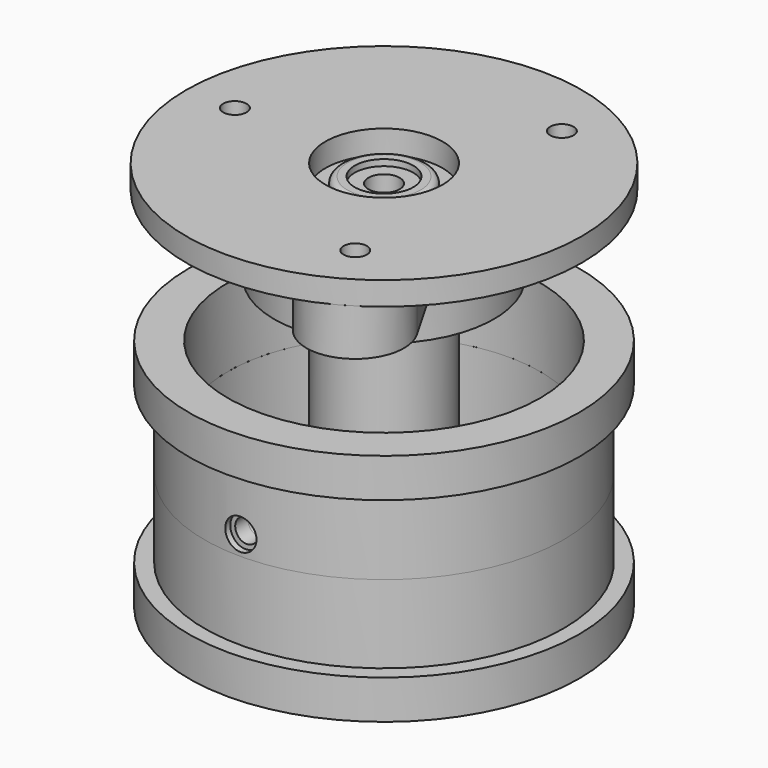
from build123d import *

# Parameters (mm, degrees)
F4_R           = 7.5
F4_R_2         = 3.75
F4_R_3         = 2.25
F5_DEPTH       = 10
F6_DEPTH       = 7.5
F9_W           = 2.45
F9_H           = 5
F11_R          = 0.2
F11_2_R        = 0.2
F12_R          = 0.6
F12_2_R        = 0.6
F13_R          = 0.8
F18_R          = 3.75
F18_R_2        = 2
F19_DEPTH      = 2
F20_DEPTH      = 6
F22_COUNT      = 3
F2_W           = 2
F2_H           = 5
F27_R          = 1.5
F28_REACH      = 54.2436406871
F31_END_RADIUS = 20
F30_R          = 3.5
F30_R_2        = 1.5
F31_REACH      = 16.9004949366
F27_R_2        = 2
F35_R          = 2
F36_DEPTH      = 47.1000001314
F38_DEPTH      = 4
F41_DEPTH      = 1
F43_R          = 25.35
F43_R_2        = 2
F43_R_3        = 7.5
F43_R_4        = 1.5
F44_DEPTH      = 3


with BuildPart() as f5:
    # F4 (on Top) → F5 (new body)
    with BuildSketch(Plane.XY):
        Circle(F4_R)
        Circle(F4_R_2, mode=Mode.SUBTRACT)
        Circle(F4_R_2)
        Circle(F4_R_3, mode=Mode.SUBTRACT)
    extrude(amount=F5_DEPTH)

    # F4 (on Top) → F6 (cut)
    with BuildSketch(Plane.XY):
        Circle(F4_R_2)
        Circle(F4_R_3, mode=Mode.SUBTRACT)
    extrude(amount=F6_DEPTH, mode=Mode.SUBTRACT)

    # F7 (on Front) → F8 (revolve)
    with BuildSketch(Plane.XZ):
        Polygon((-4.875, 12), (-6.0297005384, 10), (-3.7202994616, 10), align=None)
    revolve(axis=Axis((0, 0, 0), (0, 0, -1)))

    # F11
    f11_edges = [f5.edges().sort_by_distance(p)[0] for p in [
        (4.875, 0, 12),
    ]]
    fillet(f11_edges, radius=F11_R)

    # F12
    f12_edges = [f5.edges().sort_by_distance(p)[0] for p in [
        (-2.25, 0, 7.5),
        (-3.75, 0, 7.5),
    ]]
    fillet(f12_edges, radius=F12_R)



with BuildPart() as f10:
    # F9 (on Front) → F10 (revolve)
    with BuildSketch(Plane.XZ):
        Polygon((1.5, 20), (1.5, 10), (3.6048294078, 10), (4.875, 12.2), (6.1451705922, 10), (7.5, 10), (7.5, 35.7358983849), (5.5, 39.2), (5.5, 40), (3.95, 40), (1.5, 40), (1.5, 37), (0, 37), (0, 20), align=None)
        with Locations((2.725, 42.5)):
            Rectangle(F9_W, F9_H)
    revolve(axis=Axis((0, 0, 27.5), (0, 0, 1)))

    # F11#2
    f11_2_edges = [f10.edges().sort_by_distance(p)[0] for p in [
        (-4.875, 0, 12.2),
    ]]
    fillet(f11_2_edges, radius=F11_2_R)

    # F12#2
    f12_2_edges = [f10.edges().sort_by_distance(p)[0] for p in [
        (-1.5, 0, 20),
    ]]
    fillet(f12_2_edges, radius=F12_2_R)


with BuildPart() as f10b:
    # F9 (on Front) → F10, piece 2 (revolve)
    with BuildSketch(Plane.XZ):
        Polygon((2, 45.2), (3.95, 45.2), (3.95, 47), (5.5, 47), (5.5, 48.5), (3.75, 48.5), (3.75, 47.7), (2, 47.7), align=None)
    revolve(axis=Axis((0, 0, 27.5), (0, 0, 1)))

    # F13
    f13_edges = [f10b.edges().sort_by_distance(p)[0] for p in [
        (-5.5, 0, 48.5),
    ]]
    fillet(f13_edges, radius=F13_R)


with BuildPart() as f15:
    # F14 (on Front) → F15 (revolve)
    with BuildSketch(Plane.XZ):
        Polygon((-5.5, 40), (-5.5, 47), (-11, 47), (-11, 43.5), (-11, 40), align=None)
        Polygon((-4, 47), (-5.5, 47), (-5.5, 40), (-4, 40), (-4, 43.5), align=None)
    revolve(axis=Axis((0, 0, 43.5), (0, 0, 1)))


with BuildPart() as f17:
    # F16 (on Front) → F17 (revolve)
    with BuildSketch(Plane.XZ):
        Polygon((-7, 38.5), (-7, 40), (-11.1, 40), (-11.1, 47), (-14.1, 47), (-14.1, 44), (-14.1, 37), (-7.8660254038, 37), align=None)
    revolve(axis=Axis((0, 0, 42.5), (0, 0, -1)))

    # F18 (on face) → F19 (join)
    with BuildSketch(Plane.XY.offset(47)):
        with BuildLine():
            ThreePointArc((-13.7318717277, 3.2008903219), (-16.0131783751, 5.4345222657), (-19.1, 6.25))
            ThreePointArc((-19.1, 6.25), (-25.35, 0), (-19.1, -6.25))
            ThreePointArc((-19.1, -6.25), (-16.0131783751, -5.4345222657), (-13.7318717277, -3.2008903219))
            ThreePointArc((-13.7318717277, -3.2008903219), (-14.1, 0), (-13.7318717277, 3.2008903219))
        make_face()
        with Locations((-19.1, 0)):
            Circle(F18_R, mode=Mode.SUBTRACT)
        with Locations((-19.1, 0)):
            Circle(F18_R)
        with Locations((-19.1, 0)):
            Circle(F18_R_2, mode=Mode.SUBTRACT)
        with BuildLine():
            ThreePointArc((-13.7318717277, -3.2008903219), (-16.0131783751, -5.4345222657), (-19.1, -6.25))
            Line((-19.1, -6.25), (-12.6391257609, -6.25))
            ThreePointArc((-12.6391257609, -6.25), (-13.2733433842, -4.756927097), (-13.7318717277, -3.2008903219))
        make_face()
        with BuildLine():
            Line((-12.6391257609, 6.25), (-19.1, 6.25))
            ThreePointArc((-19.1, 6.25), (-16.0131783751, 5.4345222657), (-13.7318717277, 3.2008903219))
            ThreePointArc((-13.7318717277, 3.2008903219), (-13.2733433842, 4.756927097), (-12.6391257609, 6.25))
        make_face()
    extrude(amount=-F19_DEPTH)

    # F18 (on face) → F20 (join)
    with BuildSketch(Plane.XY.offset(47)):
        with BuildLine():
            ThreePointArc((-13.7318717277, 3.2008903219), (-16.0131783751, 5.4345222657), (-19.1, 6.25))
            ThreePointArc((-19.1, 6.25), (-25.35, 0), (-19.1, -6.25))
            ThreePointArc((-19.1, -6.25), (-16.0131783751, -5.4345222657), (-13.7318717277, -3.2008903219))
            ThreePointArc((-13.7318717277, -3.2008903219), (-14.1, 0), (-13.7318717277, 3.2008903219))
        make_face()
        with Locations((-19.1, 0)):
            Circle(F18_R, mode=Mode.SUBTRACT)
        with BuildLine():
            Line((-12.6391257609, 6.25), (-19.1, 6.25))
            ThreePointArc((-19.1, 6.25), (-16.0131783751, 5.4345222657), (-13.7318717277, 3.2008903219))
            ThreePointArc((-13.7318717277, 3.2008903219), (-13.2733433842, 4.756927097), (-12.6391257609, 6.25))
        make_face()
        with BuildLine():
            ThreePointArc((-13.7318717277, -3.2008903219), (-16.0131783751, -5.4345222657), (-19.1, -6.25))
            Line((-19.1, -6.25), (-12.6391257609, -6.25))
            ThreePointArc((-12.6391257609, -6.25), (-13.2733433842, -4.756927097), (-13.7318717277, -3.2008903219))
        make_face()
    extrude(amount=-F20_DEPTH)

    # F21: union 


with BuildPart() as f22_1:
    # F22: instance of F17
    add(f17.part.rotate(Axis((0, 0, 42.5), (0, 0, -1)), 1 * 360 / F22_COUNT))


with BuildPart() as f22_2:
    # F22: instance of F17
    add(f17.part.rotate(Axis((0, 0, 42.5), (0, 0, -1)), 2 * 360 / F22_COUNT))


with BuildPart() as f17_1:
    add(f17.part)

    # F23: union F22_2, F22_1
    add(f22_2.part)
    add(f22_1.part)


with BuildPart() as f24:
    # F1 (on Front) + F2 (on Front) → F24 (revolve)
    with BuildSketch(Plane.XZ):
        Polygon((25, 0), (25, 5), (23, 5), (23, 15), (20, 15), (20, 0), align=None)
    with BuildSketch(Plane.XZ):
        with Locations((21, 17.5)):
            Rectangle(F2_W, F2_H)
    revolve(axis=Axis((0, 0, 0), (0, 0, -1)))

    # F25: union 

    f28_end = f10.part.faces().sort_by_distance((-7.5, 0, 22.8679491924))[0]
    # F27 (on offset) → F28 (cut, up to a face of F10 that its end follows)
    with BuildSketch(Plane.XZ.offset(25)):
        with Locations((0, 17.5)):
            Circle(F27_R)
    f28_long = extrude(amount=-F28_REACH, mode=Mode.PRIVATE)
    add(split(f28_long, bisect_by=f28_end, keep=Keep.ALL, mode=Mode.PRIVATE).solids().sort_by_distance((0, -25, 17.5))[0], mode=Mode.SUBTRACT)

    f31_end = (Plane(origin=(0, 0, 10), x_dir=(-1, 0, 0), z_dir=(0, 0, -1)) * Cylinder(F31_END_RADIUS, 205.7006409456, mode=Mode.PRIVATE)).faces().sort_by_distance((-20, 0, 10))[0]
    # F30 (on offset) → F31 (join, up to the whole of a round face its end follows)
    with BuildSketch(Plane.XZ.offset(18)):
        with Locations((0, 17.5)):
            Circle(F30_R)
        with Locations((0, 17.5)):
            Circle(F30_R_2, mode=Mode.SUBTRACT)
    f31_long = extrude(amount=F31_REACH, mode=Mode.PRIVATE)
    add(split(f31_long, bisect_by=f31_end, keep=Keep.BOTTOM, mode=Mode.PRIVATE))

    # F32 (on Right) → F33 (revolve, cut)
    with BuildSketch(Plane.YZ):
        Polygon((-19, 21), (-20, 21), (-20, 20), align=None)
    revolve(axis=Axis((0, 0, 15), (0, 0, -1)), mode=Mode.SUBTRACT)


with BuildPart() as f34:
    # F3 (on Front) → F34 (revolve)
    with BuildSketch(Plane.XZ):
        Polygon((25, 30), (20, 30), (20, 20), (22.2, 20), (22.2, 15), (23, 15), (23, 25), (25, 25), align=None)
    revolve(axis=Axis((0, 0, 0), (0, 0, -1)))

    # F27 (on offset) + F35 (on offset) → F36 (cut, up to face)
    with BuildSketch(Plane.XZ.offset(25)):
        with Locations((0, 17.5)):
            Circle(F27_R_2)
        with Locations((0, 17.5)):
            Circle(F27_R, mode=Mode.SUBTRACT)
    with BuildSketch(Plane.XZ.offset(25)):
        with Locations((0, 17.5)):
            Circle(F35_R)
    extrude(amount=-F36_DEPTH, mode=Mode.SUBTRACT)


with BuildPart() as f5_1:
    add(f5.part)

    add(f24.part)  # F38 merges F24
    # F37 (on face) → F38 (join)
    with BuildSketch(Plane.XY):
        with BuildLine():
            ThreePointArc((-3.0067767078, -19.7726906067), (0, -20), (3.0067767078, -19.7726906067))
            Line((3.0067767078, -19.7726906067), (5, -5.5901699437))
            ThreePointArc((5, -5.5901699437), (0, -7.5), (-5, -5.5901699437))
            Line((-5, -5.5901699437), (-3.0067767078, -19.7726906067))
        make_face()
        with BuildLine():
            Line((7.3412291828, -1.535042047), (18.6270407205, 7.2824002909))
            ThreePointArc((18.6270407205, 7.2824002909), (17.3205080757, 10), (15.6202640127, 12.4902903159))
            Line((15.6202640127, 12.4902903159), (2.3412291828, 7.1252119908))
            ThreePointArc((2.3412291828, 7.1252119908), (6.0749164139, 4.3983395236), (7.5, 0))
            ThreePointArc((7.5, 0), (7.4602017021, -0.771615555), (7.3412291828, -1.535042047))
        make_face()
        with BuildLine():
            Line((-18.6270407205, 7.2824002909), (-7.3412291828, -1.535042047))
            ThreePointArc((-7.3412291828, -1.535042047), (-6.4951905284, 3.75), (-2.3412291828, 7.1252119908))
            Line((-2.3412291828, 7.1252119908), (-15.6202640127, 12.4902903159))
            ThreePointArc((-15.6202640127, 12.4902903159), (-17.3205080757, 10), (-18.6270407205, 7.2824002909))
        make_face()
    extrude(amount=F38_DEPTH)

    # F39: union 

    # F40 (on face) → F41 (cut)
    with BuildSketch(Plane(origin=(0, 0, 0), x_dir=(1, 0, 0), z_dir=(0, 0, -1))):
        with BuildLine():
            ThreePointArc((-18.6270407205, -7.2824002909), (-17.3205080757, -10), (-15.6202640127, -12.4902903159))
            Line((-15.6202640127, -12.4902903159), (-14.6502345253, -12.0983729631))
            ThreePointArc((-14.6502345253, -12.0983729631), (-16.4544826719, -9.5), (-17.8026155932, -6.6382887887))
            Line((-17.8026155932, -6.6382887887), (-18.6270407205, -7.2824002909))
        make_face()
        with BuildLine():
            Line((14.6502345253, -12.0983729631), (15.6202640127, -12.4902903159))
            ThreePointArc((15.6202640127, -12.4902903159), (17.3205080757, -10), (18.6270407205, -7.2824002909))
            Line((18.6270407205, -7.2824002909), (17.8026155932, -6.6382887887))
            ThreePointArc((17.8026155932, -6.6382887887), (16.4544826719, -9.5), (14.6502345253, -12.0983729631))
        make_face()
        with BuildLine():
            ThreePointArc((-8.4751793611, 0.6491030715), (-7.3612159322, -4.25), (-3.6754499309, -7.6642721641))
            Line((-3.6754499309, -7.6642721641), (-2.3412291828, -7.1252119908))
            ThreePointArc((-2.3412291828, -7.1252119908), (-6.4951905284, -3.75), (-7.3412291828, 1.535042047))
            Line((-7.3412291828, 1.535042047), (-8.4751793611, 0.6491030715))
        make_face()
        with BuildLine():
            Line((2.3412291828, -7.1252119908), (3.6754499309, -7.6642721641))
            ThreePointArc((3.6754499309, -7.6642721641), (7.1934457811, -4.5281715729), (8.5, 0))
            ThreePointArc((8.5, 0), (8.4937925737, 0.3247887243), (8.4751793611, 0.6491030715))
            Line((8.4751793611, 0.6491030715), (7.3412291828, 1.535042047))
            ThreePointArc((7.3412291828, 1.535042047), (7.4602017021, 0.771615555), (7.5, 0))
            ThreePointArc((7.5, 0), (6.0749164139, -4.3983395236), (2.3412291828, -7.1252119908))
        make_face()
        with BuildLine():
            ThreePointArc((3.0067767078, 19.7726906067), (0, 20), (-3.0067767078, 19.7726906067))
            Line((-3.0067767078, 19.7726906067), (-3.1523810679, 18.7366617518))
            ThreePointArc((-3.1523810679, 18.7366617518), (0, 19), (3.1523810679, 18.7366617518))
            Line((3.1523810679, 18.7366617518), (3.0067767078, 19.7726906067))
        make_face()
        with BuildLine():
            ThreePointArc((4.7997294302, 7.0151690926), (0, 8.5), (-4.7997294302, 7.0151690926))
            Line((-4.7997294302, 7.0151690926), (-5, 5.5901699437))
            ThreePointArc((-5, 5.5901699437), (0, 7.5), (5, 5.5901699437))
            Line((5, 5.5901699437), (4.7997294302, 7.0151690926))
        make_face()
    extrude(amount=-F41_DEPTH, mode=Mode.SUBTRACT)


with BuildPart() as f44:
    # F43 (on offset) → F44 (new body)
    with BuildSketch(Plane.XY.offset(47)):
        Circle(F43_R)
        with Locations((9.55, -16.5410852123)):
            Circle(F43_R_2, mode=Mode.SUBTRACT)
        with Locations((-19.1, 0)):
            Circle(F43_R_2, mode=Mode.SUBTRACT)
        Circle(F43_R_3, mode=Mode.SUBTRACT)
        with Locations((9.55, 16.5410852123)):
            Circle(F43_R_2, mode=Mode.SUBTRACT)
        with Locations((-19.1, 0)):
            Circle(F43_R_2)
        with Locations((-19.1, 0)):
            Circle(F43_R_4, mode=Mode.SUBTRACT)
        with Locations((9.55, -16.5410852123)):
            Circle(F43_R_2)
        with Locations((9.55, -16.5410852123)):
            Circle(F43_R_4, mode=Mode.SUBTRACT)
        with Locations((9.55, 16.5410852123)):
            Circle(F43_R_2)
        with Locations((9.55, 16.5410852123)):
            Circle(F43_R_4, mode=Mode.SUBTRACT)
    extrude(amount=F44_DEPTH)


solid = Compound([f10.part, f10b.part, f15.part, f17_1.part, f34.part, f5_1.part, f44.part])
